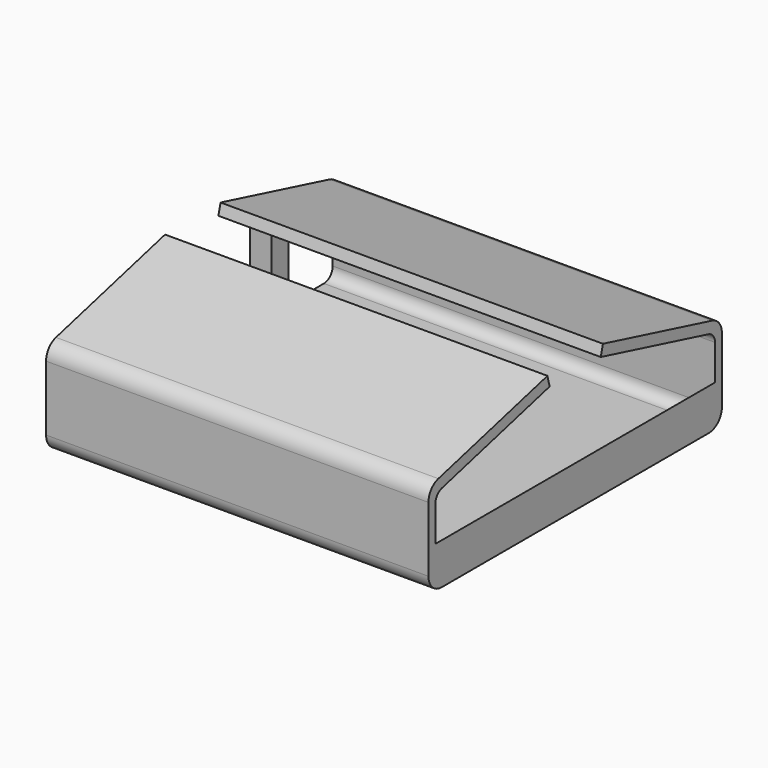
from build123d import *

# Parameters (mm, degrees)
F1_DEPTH = 88.9
F3_DEPTH = 5
F4_W     = 81.28
F4_H     = 7.62
F5_DEPTH = 7.62
F6_R     = 3.81
F7_R     = 2.54
F8_SIZE  = 7.61999


# Not quite as in the source:
# - a fillet or chamfer is up to 0.001 mm smaller than in the source, because OpenCascade refuses the exact size


with BuildPart() as f1:
    # F0 (on Right) → F1 (new body)
    with BuildSketch(Plane.YZ):
        Polygon((17.24, 2), (17.24, 0), (59.88, 0), (59.88, 21.8881247946), (25.3046089437, 30.7845262293), (24.6716719012, 28.3246500739), (57.88, 19.78), (57.88, 2), align=None)
        Polygon((-25.4, 21.8881247946), (-25.4, 0), (17.24, 0), (17.24, 2), (-23.4, 2), (-23.4, 19.78), (9.8083280988, 28.3246500739), (9.1753910563, 30.7845262293), align=None)
    extrude(amount=F1_DEPTH)

    # F2 (on Right) → F3 (join)
    with BuildSketch(Plane.YZ):
        Polygon((33.83, 2), (38.83, 2), (38.83, 17.7), (38.83, 24.6816494725), (33.83, 25.9681716437), (33.83, 17.7), align=None)
        Polygon((-4.35, 17.7), (-4.35, 2), (0.65, 2), (0.65, 17.7), (0.65, 25.9681716437), (-4.35, 24.6816494725), align=None)
    extrude(amount=F3_DEPTH)

    # F4 (on face) → F5 (join)
    with BuildSketch(Plane.YZ.offset(88.9)):
        with Locations((17.24, 5.81)):
            Rectangle(F4_W, F4_H)
    extrude(amount=-F5_DEPTH)

    # F6
    f6_edges = [f1.edges().sort_by_distance(p)[0] for p in [
        (44.45, -25.4, 0),
        (44.45, 59.88, 0),
        (44.45, -25.4, 21.888125),
        (44.45, 59.88, 21.888125),
    ]]
    fillet(f6_edges, radius=F6_R)

    # F7
    f7_edges = [f1.edges().sort_by_distance(p)[0] for p in [
        (40.64, 57.88, 2),
        (40.64, -23.4, 2),
        (44.45, -23.4, 19.78),
        (44.45, 57.88, 19.78),
    ]]
    fillet(f7_edges, radius=F7_R)

    # F8 (size 7.62 in the source; OpenCascade refuses exactly that, so slightly less here)
    f8_edges = [f1.edges().sort_by_distance(p)[0] for p in [
        (81.28, 17.24, 9.62),
    ]]
    chamfer(f8_edges, length=F8_SIZE)


solid = f1.part
